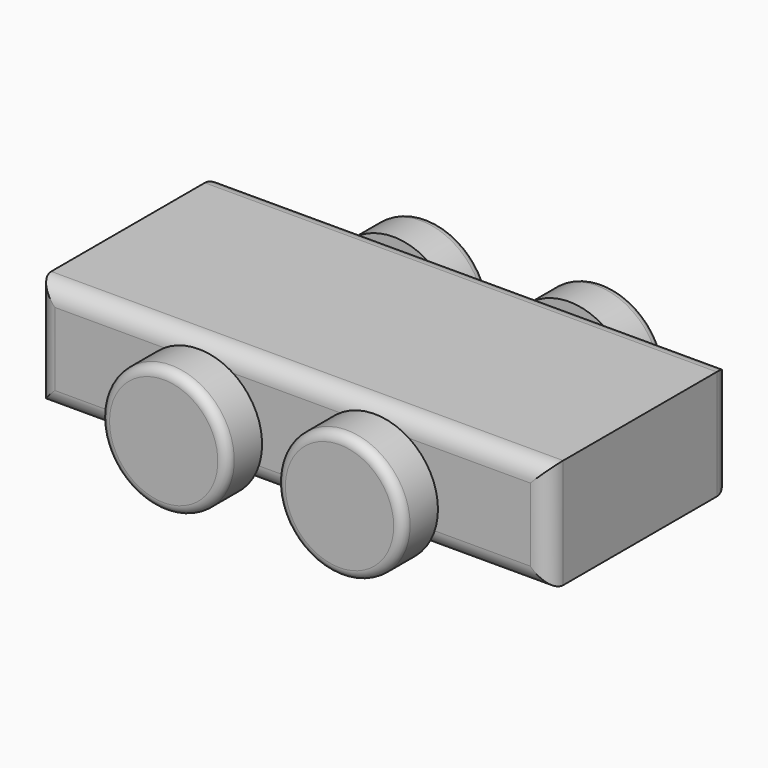
from build123d import *

# Parameters (mm, degrees)
F1_W     = 177.8
F1_H     = 38.1
F3_DEPTH = 39.6875
F5_R     = 21.9796121182
F6_DEPTH = 15.24
F7_R     = 3.175
F8_R     = 6.35


# Not quite as in the source:
# - the program builds the solid bodies; features that only make, move or delete a surface that nothing else refers to are left out


with BuildPart() as f3:
    # F1 (on face) → F3 (new body, symmetric)
    with BuildSketch(Plane.XZ):
        Rectangle(F1_W, F1_H)
    extrude(amount=F3_DEPTH, both=True)

    # F8
    f8_edges = [f3.edges().sort_by_distance(p)[0] for p in [
        (0, -39.6875, 19.05),
        (-88.9, -39.6875, 0),
        (0, -39.6875, -19.05),
        (88.9, -39.6875, 0),
        (88.9, 39.6875, 0),
        (0, 39.6875, 19.05),
        (0, 39.6875, -19.05),
        (-88.9, 39.6875, 0),
    ]]
    fillet(f8_edges, radius=F8_R)


with BuildPart() as f6:
    # F5 (on offset) → F6 (new body)
    with BuildSketch(Plane.XZ.offset(42.2275)):
        with Locations((30.5357445031, -4.0553878818)):
            Circle(F5_R)
    extrude(amount=F6_DEPTH)

    # F7
    f7_edges = [f6.edges().sort_by_distance(p)[0] for p in [
        (8.556132, -57.4675, -4.055388),
    ]]
    fillet(f7_edges, radius=F7_R)


with BuildPart() as f9_1:
    # F9: instance of F6
    add(f6.part.mirror(Plane.XZ))


with BuildPart() as f10_1:
    # F10: instance of F6
    add(f6.part.mirror(Plane.YZ))


with BuildPart() as f10_2:
    # F10: instance of F9_1
    add(f9_1.part.mirror(Plane.YZ))


solid = Compound([f3.part, f6.part, f9_1.part, f10_1.part, f10_2.part])
